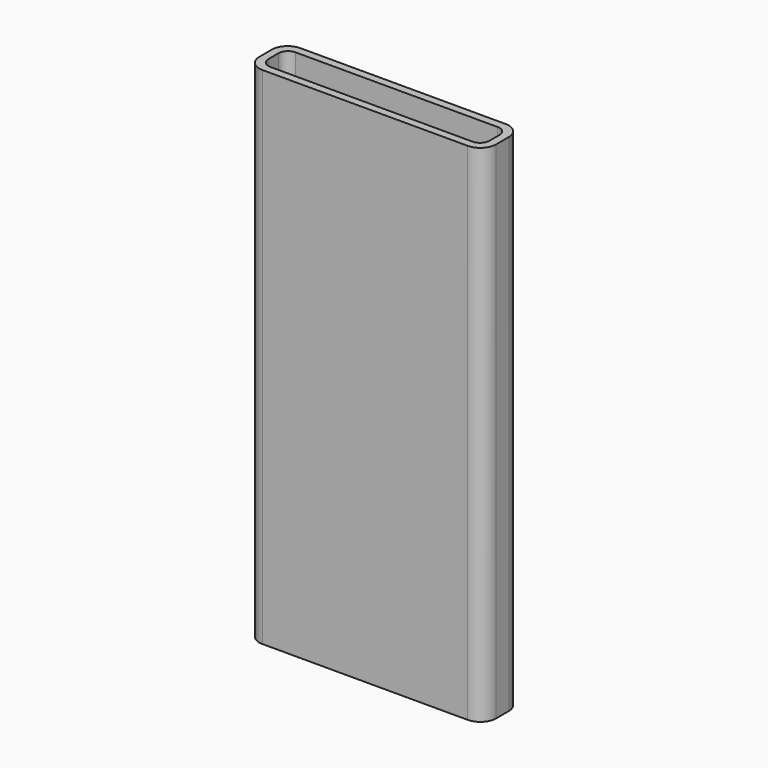
from build123d import *

# Parameters (mm, degrees)
F0_W     = 75
F0_H     = 15
F1_DEPTH = 5
F2_W     = 75
F2_H     = 15
F2_W_2   = 70
F2_H_2   = 10
F3_DEPTH = 160
F4_R     = 5
F5_R     = 5
F6_R     = 5
F7_R     = 5
F8_R     = 3
F9_R     = 3
F10_R    = 3
F11_R    = 3
F12_R    = 3


# Not quite as in the source:
# - two fillets or chamfers of one size are made in one step


with BuildPart() as f1:
    # F0 (on Top) → F1 (new body)
    with BuildSketch(Plane.XY):
        with Locations((-35, 5)):
            Rectangle(F0_W, F0_H)
    extrude(amount=F1_DEPTH)

    # F2 (on face) → F3 (join)
    with BuildSketch(Plane(origin=(0, 0, 0), x_dir=(1, 0, 0), z_dir=(0, 0, -1))):
        with Locations((-35, -5)):
            Rectangle(F2_W, F2_H)
        with Locations((-35, -5)):
            Rectangle(F2_W_2, F2_H_2, mode=Mode.SUBTRACT)
    extrude(amount=-F3_DEPTH)

    # F4
    f4_edges = [f1.edges().sort_by_distance(p)[0] for p in [
        (-72.5, 12.5, 80),
    ]]
    fillet(f4_edges, radius=F4_R)

    # F5
    f5_edges = [f1.edges().sort_by_distance(p)[0] for p in [
        (-72.5, -2.5, 80),
    ]]
    fillet(f5_edges, radius=F5_R)

    # F6
    f6_edges = [f1.edges().sort_by_distance(p)[0] for p in [
        (2.5, -2.5, 80),
    ]]
    fillet(f6_edges, radius=F6_R)

    # F7
    f7_edges = [f1.edges().sort_by_distance(p)[0] for p in [
        (2.5, 12.5, 80),
    ]]
    fillet(f7_edges, radius=F7_R)

    # F8
    f8_edges = [f1.edges().sort_by_distance(p)[0] for p in [
        (-70, 10, 82.5),
    ]]
    fillet(f8_edges, radius=F8_R)

    # F9
    f9_edges = [f1.edges().sort_by_distance(p)[0] for p in [
        (0, 10, 82.5),
    ]]
    fillet(f9_edges, radius=F9_R)

    # F10
    f10_edges = [f1.edges().sort_by_distance(p)[0] for p in [
        (-70, 0, 82.5),
    ]]
    fillet(f10_edges, radius=F10_R)

    # F11
    f11_edges = [f1.edges().sort_by_distance(p)[0] for p in [
        (0, 0, 82.5),
    ]]
    fillet(f11_edges, radius=F11_R)

    # F12
    f12_edges = [f1.edges().sort_by_distance(p)[0] for p in [
        (-35, 0, 5),
        (-0.87868, 0.87868, 5),
        (-69.12132, 0.87868, 5),
        (0, 5, 5),
        (-70, 5, 5),
        (-0.87868, 9.12132, 5),
        (-69.12132, 9.12132, 5),
        (-35, 10, 5),
    ]]
    fillet(f12_edges, radius=F12_R)


solid = f1.part
